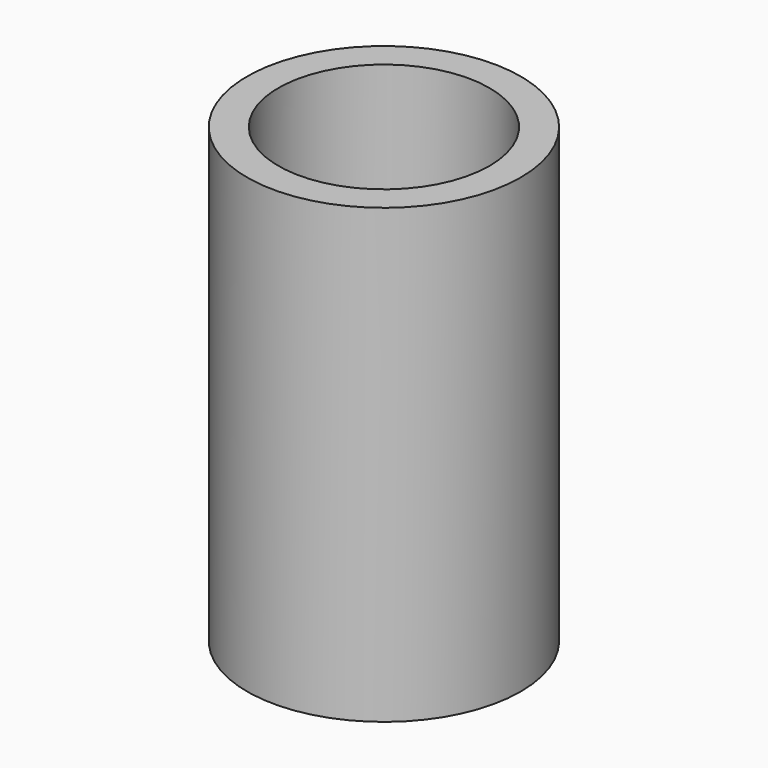
from build123d import *

# Parameters (mm, degrees)
F0_R          = 39.2481285359
F0_R_2        = 30.2795361801
F1_DEPTH      = 60.19936
F1_DEPTH_BACK = 69.6123


# Not quite as in the source:
# - a feature of the source that left no trace in its solid (it failed there, or was rolled back) is left out


with BuildPart() as f1:
    # F0 (on Top) → F1 (new body, two sides)
    with BuildSketch(Plane.XY) as f1_sk:
        Circle(F0_R)
        Circle(F0_R_2, mode=Mode.SUBTRACT)
    extrude(amount=F1_DEPTH)
    extrude(f1_sk.sketch, amount=-F1_DEPTH_BACK)


solid = f1.part
